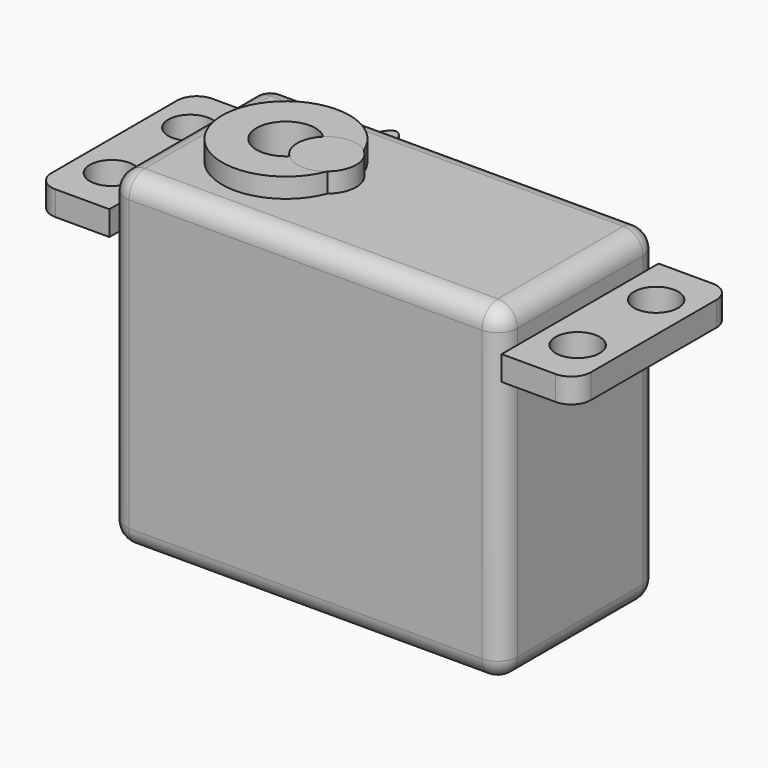
from build123d import *

# Parameters (mm, degrees)
F0_W      = 7.5
F0_H      = 20
F0_R      = 2.25
F1_DEPTH  = 2.5
F0_W_2    = 40
F0_R_2    = 6.5
F2_DEPTH  = 6
F0_R_3    = 3
F3_DEPTH  = 27.5
F4_DEPTH  = 8
F5_R      = 2
F5_2_R    = 2
F5_3_R    = 2
F7_R      = 0.75
F8_DEPTH  = 3
F9_DEPTH  = 3
F11_R     = 3
F12_DEPTH = 8


# Not quite as in the source:
# - a feature of the source that left no trace in its solid (it failed there, or was rolled back) is left out


with BuildPart() as f1:
    # F0 (on Top) → F1 (new body)
    with BuildSketch(Plane.XY):
        with Locations((23.75, 0)):
            Rectangle(F0_W, F0_H)
        with Locations((23.75, -5)):
            Circle(F0_R, mode=Mode.SUBTRACT)
        with Locations((23.75, 5)):
            Circle(F0_R, mode=Mode.SUBTRACT)
    extrude(amount=F1_DEPTH)

    # F5
    f5_edges = [f1.edges().sort_by_distance(p)[0] for p in [
        (27.5, -10, 1.25),
        (27.5, 10, 1.25),
    ]]
    fillet(f5_edges, radius=F5_R)


with BuildPart() as f1b:
    # F0 (on Top) → F1, piece 2 (new body)
    with BuildSketch(Plane.XY):
        with Locations((-23.75, 0)):
            Rectangle(F0_W, F0_H)
        with Locations((-23.75, -5)):
            Circle(F0_R, mode=Mode.SUBTRACT)
        with Locations((-23.75, 5)):
            Circle(F0_R, mode=Mode.SUBTRACT)
    extrude(amount=F1_DEPTH)

    # F5#2
    f5_2_edges = [f1b.edges().sort_by_distance(p)[0] for p in [
        (-27.5, -10, 1.25),
        (-27.5, 10, 1.25),
    ]]
    fillet(f5_2_edges, radius=F5_2_R)


with BuildPart() as f2:
    # F0 (on Top) → F2 (new body)
    with BuildSketch(Plane.XY):
        Rectangle(F0_W_2, F0_H)
        with Locations((-10, 0)):
            Circle(F0_R_2, mode=Mode.SUBTRACT)
    extrude(amount=F2_DEPTH)

    # F0 (on Top) → F3 (join)
    with BuildSketch(Plane.XY):
        Rectangle(F0_W_2, F0_H)
        with Locations((-10, 0)):
            Circle(F0_R_2, mode=Mode.SUBTRACT)
        with Locations((-10, 0)):
            Circle(F0_R_2)
        with Locations((-10, 0)):
            Circle(F0_R_3, mode=Mode.SUBTRACT)
    extrude(amount=-F3_DEPTH)

    # F0 (on Top) → F4 (join)
    with BuildSketch(Plane.XY):
        with Locations((-10, 0)):
            Circle(F0_R_2)
        with Locations((-10, 0)):
            Circle(F0_R_3, mode=Mode.SUBTRACT)
    extrude(amount=F4_DEPTH)

    # F5#3
    f5_3_edges = [f2.edges().sort_by_distance(p)[0] for p in [
        (0, -10, 6),
        (0, 10, 6),
        (0, 10, -27.5),
        (0, -10, -27.5),
        (-20, 10, -10.75),
        (-20, -10, -10.75),
        (20, -10, -10.75),
        (20, 10, -10.75),
        (20, 0, -27.5),
        (20, 0, 6),
        (-20, 0, 6),
        (-20, 0, -27.5),
    ]]
    fillet(f5_3_edges, radius=F5_3_R)


with BuildPart() as f8:
    # F7 (on Top) → F8 (new body)
    with BuildSketch(Plane.XY):
        with BuildLine():
            ThreePointArc((-13, 0), (-10, -3), (-7, 0))
            ThreePointArc((-7, 0), (-10, 3), (-13, 0))
        make_face()
        with BuildLine():
            ThreePointArc((-13, 0), (-10, 3), (-7, 0))
            add(Edge.make_bspline(
                [(-13, 0), (-13, 7), (-10, 21), (-7, 7), (-7, 0)],
                knots=[0, 0, 0, 0, 0.5, 1, 1, 1, 1], degree=3))
        make_face()
        with Locations((-10, 5.5)):
            Circle(F7_R, mode=Mode.SUBTRACT)
        with Locations((-10, 7.5)):
            Circle(F7_R, mode=Mode.SUBTRACT)
        with Locations((-10, 9.5)):
            Circle(F7_R, mode=Mode.SUBTRACT)
        with Locations((-10, 11.5)):
            Circle(F7_R, mode=Mode.SUBTRACT)
    extrude(amount=F8_DEPTH)


with BuildPart() as f9:
    # F7 (on Top) → F9 (new body)
    with BuildSketch(Plane.XY):
        with BuildLine():
            ThreePointArc((-13, 0), (-10, -3), (-7, 0))
            ThreePointArc((-7, 0), (-10, 3), (-13, 0))
        make_face()
        with BuildLine():
            ThreePointArc((-13, 0), (-10, 3), (-7, 0))
            add(Edge.make_bspline(
                [(-13, 0), (-13, 7), (-10, 21), (-7, 7), (-7, 0)],
                knots=[0, 0, 0, 0, 0.5, 1, 1, 1, 1], degree=3))
        make_face()
        with Locations((-10, 5.5)):
            Circle(F7_R, mode=Mode.SUBTRACT)
        with Locations((-10, 7.5)):
            Circle(F7_R, mode=Mode.SUBTRACT)
        with Locations((-10, 9.5)):
            Circle(F7_R, mode=Mode.SUBTRACT)
        with Locations((-10, 11.5)):
            Circle(F7_R, mode=Mode.SUBTRACT)
    extrude(amount=F9_DEPTH)


with BuildPart() as f12:
    # F11 (on Top) → F12 (new body)
    with BuildSketch(Plane.XY):
        with Locations((-5.8363600008, 0)):
            Circle(F11_R)
    extrude(amount=F12_DEPTH)


solid = Compound([f1.part, f1b.part, f2.part, f8.part, f12.part])
